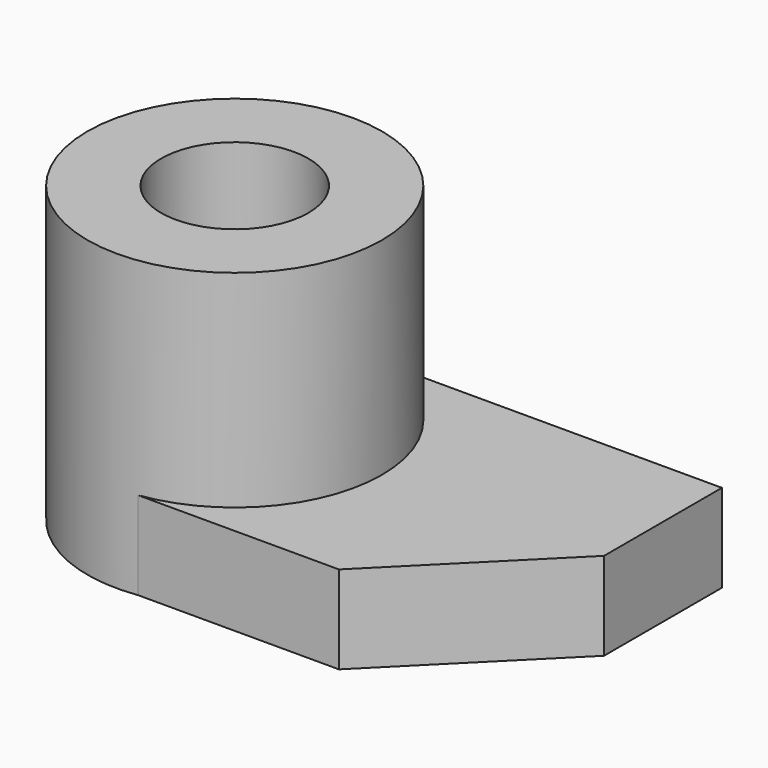
from build123d import *

# Parameters (mm, degrees)
F2_DEPTH = 50.8
F1_R     = 12.7
F3_DEPTH = 50.8
F4_R     = 25.4
F4_R_2   = 12.7
F5_DEPTH = 50.8


# Not quite as in the source:
# - ends of sketch curves that miss each other by under 0.0002 mm in the source are joined


with BuildPart() as f2:
    # F0 (on Front) → F2 (new body)
    with BuildSketch(Plane.XZ):
        Polygon((0, 15.1726854965), (0, 0), (88.9, 0), (88.9, 15.1726854965), (38.1, 15.1726854965), align=None)
    extrude(amount=-F2_DEPTH)

    # F1 (on Top) → F3 (intersect)
    with BuildSketch(Plane.XY):
        with BuildLine():
            ThreePointArc((25.4023582082, 0), (43.3628704503, 7.4394877579), (50.8023582082, 25.4))
            ThreePointArc((50.8023582082, 25.4), (50.8017686493, 25.5730584989), (50.8, 25.7461089641))
            ThreePointArc((50.8, 25.7461089641), (43.2400827311, 43.4824661992), (25.4023582082, 50.8))
            ThreePointArc((25.4023582082, 50.8), (25.4011791041, 50.7999999726), (25.4, 50.7999998905))
            ThreePointArc((25.4, 50.7999998905), (0.0023582082, 25.4), (25.4, 1.095e-07))
            ThreePointArc((25.4, 1.095e-07), (25.4011791041, 2.74e-08), (25.4023582082, 0))
        make_face()
        with Locations((25.4023582082, 25.4)):
            Circle(F1_R, mode=Mode.SUBTRACT)
        with BuildLine():
            ThreePointArc((50.8, 25.7461089641), (50.8017686493, 25.5730584989), (50.8023582082, 25.4))
            ThreePointArc((50.8023582082, 25.4), (43.3628704503, 7.4394877579), (25.4023582082, 0))
            Line((25.4023582082, 0), (51.1508577362, 0))
            Line((51.1508577362, 0), (63.5, 0))
            Line((63.5, 0), (88.9, 25.4))
            Line((88.9, 25.4), (88.9, 50.8))
            Line((88.9, 50.8), (50.4585755345, 50.8))
            Line((50.4585755345, 50.8), (25.4023582082, 50.8))
            ThreePointArc((25.4023582082, 50.8), (43.2400827311, 43.4824661992), (50.8, 25.7461089641))
        make_face()
        with BuildLine():
            ThreePointArc((0, 25.4), (7.4394877579, 7.4394877579), (25.4, 0))
            ThreePointArc((25.4, 0), (0.0023582082, 25.4), (25.4, 50.7999998905))
            ThreePointArc((25.4, 50.7999998905), (7.4394877579, 43.3605122421), (0, 25.4))
        make_face()
    extrude(amount=F3_DEPTH, mode=Mode.INTERSECT)

    # F4 (on Top) → F5 (join)
    with BuildSketch(Plane.XY):
        with Locations((25.4, 25.1621566713)):
            Circle(F4_R)
        with Locations((25.4, 25.1621566713)):
            Circle(F4_R_2, mode=Mode.SUBTRACT)
    extrude(amount=F5_DEPTH)


solid = f2.part
